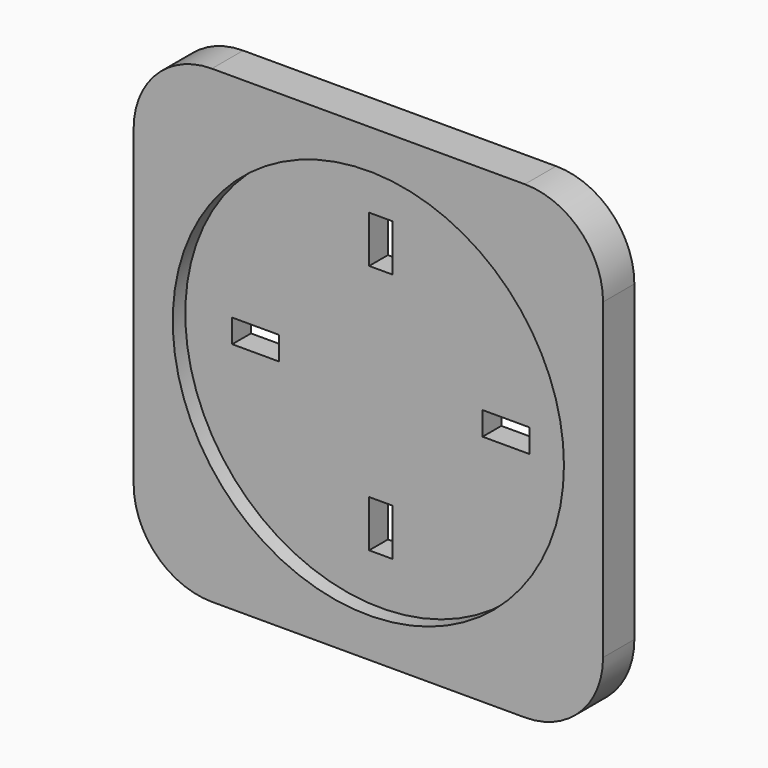
from build123d import *

# Parameters (mm, degrees)
F0_W            = 60
F0_H            = 60
F1_DEPTH        = 5
F2_R            = 25
F3_DEPTH        = 2
F4_R            = 10
F5_R            = 10
F6_R            = 10
F7_R            = 10
F8_W            = 3
F8_H            = 6
F9_DEPTH        = 3.001
F9_COPIES_COUNT = 4


# Not quite as in the source:
# - a pattern or mirror of a feature is missing from the dataset's text; its kind, count and spacing are read off the source's solid


with BuildPart() as f1:
    # F0 (on Front) → F1 (new body)
    with BuildSketch(Plane.XZ):
        Rectangle(F0_W, F0_H)
    extrude(amount=F1_DEPTH)

    # F2 (on face) → F3 (cut)
    with BuildSketch(Plane.XZ.offset(5)):
        Circle(F2_R)
    extrude(amount=-F3_DEPTH, mode=Mode.SUBTRACT)

    # F4
    f4_edges = [f1.edges().sort_by_distance(p)[0] for p in [
        (-30, -2.5, 30),
    ]]
    fillet(f4_edges, radius=F4_R)

    # F5
    f5_edges = [f1.edges().sort_by_distance(p)[0] for p in [
        (30, -2.5, 30),
    ]]
    fillet(f5_edges, radius=F5_R)

    # F6
    f6_edges = [f1.edges().sort_by_distance(p)[0] for p in [
        (-30, -2.5, -30),
    ]]
    fillet(f6_edges, radius=F6_R)

    # F7
    f7_edges = [f1.edges().sort_by_distance(p)[0] for p in [
        (30, -2.5, -30),
    ]]
    fillet(f7_edges, radius=F7_R)

    # F8 (on face) → F9 (cut, through all)
    with BuildSketch(Plane.XZ.offset(3)):
        with Locations((0, 16)):
            Rectangle(F8_W, F8_H)
    f9 = extrude(amount=-F9_DEPTH, mode=Mode.SUBTRACT)

    # F9_copies: F9 ×4 about axis
    f9_copies_axis = Axis((0, 0, 0), (0, 1, 0))
    for i in range(1, F9_COPIES_COUNT):
        add(f9.rotate(f9_copies_axis, i * 360 / F9_COPIES_COUNT), mode=Mode.SUBTRACT)


solid = f1.part
